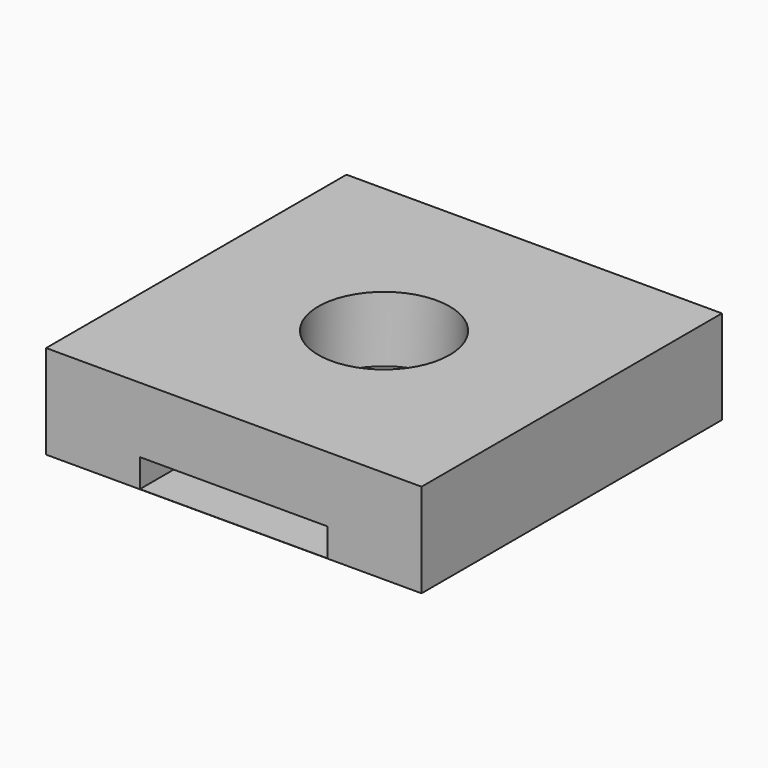
from build123d import *

# Parameters (mm, degrees)
F0_W     = 20
F0_H     = 20
F0_R     = 3.5
F1_DEPTH = 5
F2_W     = 10
F2_H     = 1.5
F3_DEPTH = 12.5


# Not quite as in the source:
# - a feature names something its author has since deleted; it is built from what else it names


with BuildPart() as f1:
    # F0 (on Top) → F1 (new body)
    with BuildSketch(Plane.XY):
        Rectangle(F0_W, F0_H)
        Circle(F0_R, mode=Mode.SUBTRACT)
    extrude(amount=F1_DEPTH)

    # F2 (on Front) → F3 (cut, symmetric)
    with BuildSketch(Plane.XZ):
        with Locations((0, 0.7610858302)):
            Rectangle(F2_W, F2_H)
    extrude(amount=F3_DEPTH, both=True, mode=Mode.SUBTRACT)


solid = f1.part
